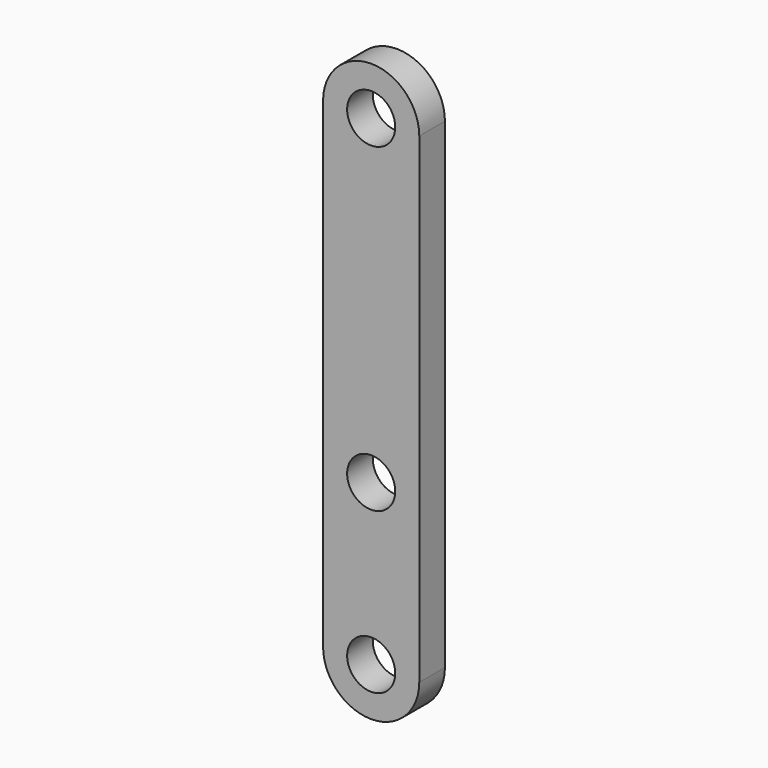
from build123d import *

# Parameters (mm, degrees)
F1_DEPTH = 10
F2_R     = 7.5
F3_DEPTH = 25


# Not quite as in the source:
# - a feature names something its author has since deleted; it is built from what else it names


with BuildPart() as f1:
    # F0 (on Front) → F1 (new body)
    with BuildSketch(Plane.XZ):
        with BuildLine():
            Line((15, -75), (15, 75))
            ThreePointArc((15, 75), (0, 90), (-15, 75))
            Line((-15, 75), (-15, -75))
            ThreePointArc((-15, -75), (0, -90), (15, -75))
        make_face()
    extrude(amount=F1_DEPTH)

    # F2 (on face) → F3 (cut, symmetric)
    with BuildSketch(Plane.XZ.offset(10)):
        with Locations((0, 75)):
            Circle(F2_R)
        with Locations((0, -75)):
            Circle(F2_R)
        with Locations((0, -25)):
            Circle(F2_R)
    extrude(amount=F3_DEPTH, both=True, mode=Mode.SUBTRACT)


solid = f1.part
